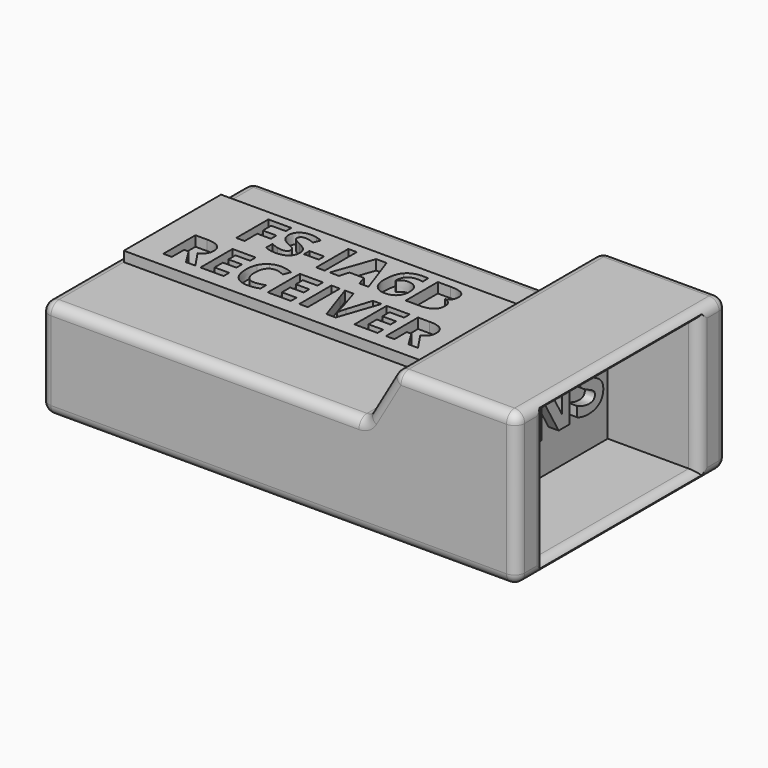
from build123d import *

# Parameters (mm, degrees)
F0_W          = 47
F0_H          = 15
F1_DEPTH      = 26
F3_DEPTH      = 26.001
F5_DEPTH      = 9
F6_TEXT_SIZE  = 6.9444444444
F7_DEPTH      = 1
F8_T1_DEPTH   = 26
F8_T3_DEPTH   = 30.4226497308
F8_T5_DEPTH   = 24
F8_T7_DEPTH   = 7.8038475773
F8_T9_DEPTH   = 13
F8_T11_DEPTH  = 45
F8_T13_DEPTH  = 4.8452994616
F8_T15_DEPTH  = 10.4226497308
F8_T17_DEPTH  = 19
F8_S21_W      = 1.02
F8_S21_H      = 1.02
F8_T22_DEPTH  = 1.02
F8_S27_W      = 1.02
F8_S27_H      = 1.02
F8_T28_DEPTH  = 1.02
F8_S33_W      = 1.02
F8_S33_H      = 1.02
F8_T34_DEPTH  = 1.02
F8_S39_W      = 1.02
F8_S39_H      = 1.02
F8_T40_DEPTH  = 1.02
F8_S45_W      = 1.02
F8_S45_H      = 1.02
F8_T46_DEPTH  = 1.02
F8_S51_W      = 1.02
F8_S51_H      = 1.02
F8_T52_DEPTH  = 1.02
F8_T58_DEPTH  = 1.02
F8_S63_W      = 1.02
F8_S63_H      = 1.02
F8_T64_DEPTH  = 1.02
F8_S69_W      = 1.02
F8_S69_H      = 1.02
F8_T70_DEPTH  = 1.02
F8_T76_DEPTH  = 1.02
F8_T80_ANGLE  = 60
F8_T82_ANGLE  = 60
F8_T87_DEPTH  = 21.5
F8_T91_DEPTH  = 15.5
F8_T99_DEPTH  = 21.5
F8_T103_DEPTH = 15.5
F8_T111_DEPTH = 15.5
F8_T116_DEPTH = 21.5
F8_T123_DEPTH = 21.5
F8_T127_DEPTH = 15.5
F9_W          = 0.8411458333
F9_H          = 3.9661458333
F9_W_2        = 1.4565972222
F9_H_2        = 0.6779513889
F10_DEPTH     = 1


# Not quite as in the source:
# - a fillet or chamfer that OpenCascade refuses, or shapes differently, is made with other operations: its cross-section is extruded or revolved along the edge and cut away or added
# - Text() gives the source's letters only with a copy of the font that has no kerning and outlines rounded to 1/6400 em; it was checked with that copy


with BuildPart() as f1:
    # F0 (on Front) → F1 (new body)
    with BuildSketch(Plane.XZ):
        with Locations((23.5, -7.5)):
            Rectangle(F0_W, F0_H)
    extrude(amount=F1_DEPTH)

    # F2 (on face) → F3 (cut, through all)
    with BuildSketch(Plane.XZ.offset(26)):
        Polygon((0, 0), (0, -5.1961524227), (32, -5.1961524227), (35, 0), align=None)
    extrude(amount=-F3_DEPTH, mode=Mode.SUBTRACT)

    # F4 (on face) → F5 (cut)
    with BuildSketch(Plane.YZ.offset(47)):
        Polygon((-16.9174801558, -1), (-22.5, -1), (-22.5, -9.4061652198), (-22.5, -14), (-8.8980188593, -14), (-3.5, -14), (-3.5, -5.7331291027), (-3.5, -1), align=None)
    extrude(amount=-F5_DEPTH, mode=Mode.SUBTRACT)

    # F8: fillet of radius 1 on 22 edges, made by hand

    # F8_s2 → F8_t1 (join)
    with BuildSketch(Plane.XZ):
        with BuildLine():
            ThreePointArc((32.2886751346, -4.6961524227), (31.9226497308, -5.0621778265), (31.4226497308, -5.1961524227))
            Line((31.4226497308, -5.1961524227), (32, -5.1961524227))
            Line((32, -5.1961524227), (32.2886751346, -4.6961524227))
        make_face()
    extrude(amount=F8_T1_DEPTH)

    # F8_s4 → F8_t3 (cut)
    with BuildSketch(Plane.YZ.offset(1)):
        with BuildLine():
            ThreePointArc((-26, -6.1961524227), (-25.7071067812, -5.4890456415), (-25, -5.1961524227))
            Line((-25, -5.1961524227), (-26, -5.1961524227))
            Line((-26, -5.1961524227), (-26, -6.1961524227))
        make_face()
        with BuildLine():
            ThreePointArc((0, -6.1961524227), (-0.2928932188, -5.4890456415), (-1, -5.1961524227))
            Line((-1, -5.1961524227), (0, -5.1961524227))
            Line((0, -5.1961524227), (0, -6.1961524227))
        make_face()
    extrude(amount=F8_T3_DEPTH, mode=Mode.SUBTRACT)

    # F8_s6 → F8_t5 (cut)
    with BuildSketch(Plane.XZ.offset(1)):
        with BuildLine():
            ThreePointArc((0, -6.1961524227), (0.2928932188, -5.4890456415), (1, -5.1961524227))
            Line((1, -5.1961524227), (0, -5.1961524227))
            Line((0, -5.1961524227), (0, -6.1961524227))
        make_face()
        with BuildLine():
            ThreePointArc((1, -15), (0.2928932188, -14.7071067812), (0, -14))
            Line((0, -14), (0, -15))
            Line((0, -15), (1, -15))
        make_face()
        with BuildLine():
            ThreePointArc((47, -14), (46.7071067812, -14.7071067812), (46, -15))
            Line((46, -15), (47, -15))
            Line((47, -15), (47, -14))
        make_face()
        with BuildLine():
            ThreePointArc((46, 0), (46.7071067812, -0.2928932188), (47, -1))
            Line((47, -1), (47, 0))
            Line((47, 0), (46, 0))
        make_face()
        with BuildLine():
            ThreePointArc((35.5773502692, 0), (35.0773502692, -0.1339745962), (34.7113248654, -0.5))
            Line((34.7113248654, -0.5), (35, 0))
            Line((35, 0), (35.5773502692, 0))
        make_face()
    extrude(amount=F8_T5_DEPTH, mode=Mode.SUBTRACT)

    # F8_s8 → F8_t7 (cut)
    with BuildSketch(Plane.XY.offset(-14)):
        with BuildLine():
            ThreePointArc((1, 0), (0.2928932188, -0.2928932188), (0, -1))
            Line((0, -1), (0, 0))
            Line((0, 0), (1, 0))
        make_face()
        with BuildLine():
            ThreePointArc((1, -26), (0.2928932188, -25.7071067812), (0, -25))
            Line((0, -25), (0, -26))
            Line((0, -26), (1, -26))
        make_face()
    extrude(amount=F8_T7_DEPTH, mode=Mode.SUBTRACT)

    # F8_s10 → F8_t9 (cut)
    with BuildSketch(Plane.XY.offset(-14)):
        with BuildLine():
            ThreePointArc((46, 0), (46.7071067812, -0.2928932188), (47, -1))
            Line((47, -1), (47, 0))
            Line((47, 0), (46, 0))
        make_face()
        with BuildLine():
            ThreePointArc((46, -26), (46.7071067812, -25.7071067812), (47, -25))
            Line((47, -25), (47, -26))
            Line((47, -26), (46, -26))
        make_face()
        with BuildLine():
            ThreePointArc((47, -2.5), (46.7071067812, -3.2071067812), (46, -3.5))
            Line((46, -3.5), (47, -3.5))
            Line((47, -3.5), (47, -2.5))
        make_face()
        with BuildLine():
            ThreePointArc((47, -23.5), (46.7071067812, -22.7928932188), (46, -22.5))
            Line((46, -22.5), (47, -22.5))
            Line((47, -22.5), (47, -23.5))
        make_face()
    extrude(amount=F8_T9_DEPTH, mode=Mode.SUBTRACT)

    # F8_s12 → F8_t11 (cut)
    with BuildSketch(Plane.YZ.offset(1)):
        with BuildLine():
            ThreePointArc((0, -14), (-0.2928932188, -14.7071067812), (-1, -15))
            Line((-1, -15), (0, -15))
            Line((0, -15), (0, -14))
        make_face()
        with BuildLine():
            ThreePointArc((-26, -14), (-25.7071067812, -14.7071067812), (-25, -15))
            Line((-25, -15), (-26, -15))
            Line((-26, -15), (-26, -14))
        make_face()
    extrude(amount=F8_T11_DEPTH, mode=Mode.SUBTRACT)

    # F8_s14 → F8_t13 (cut)
    with BuildSketch(Plane(origin=(6.0386751346, 0, 10.4592921435), x_dir=(0, 1, 0), z_dir=(0.5, 0, 0.8660254038))):
        with BuildLine():
            ThreePointArc((0, -31.3108891325), (-0.2928932188, -30.6037823513), (-1, -30.3108891325))
            Line((-1, -30.3108891325), (0, -30.3108891325))
            Line((0, -30.3108891325), (0, -31.3108891325))
        make_face()
        with BuildLine():
            ThreePointArc((-25, -30.3108891325), (-25.7071067812, -30.6037823513), (-26, -31.3108891325))
            Line((-26, -31.3108891325), (-26, -30.3108891325))
            Line((-26, -30.3108891325), (-25, -30.3108891325))
        make_face()
    extrude(amount=F8_T13_DEPTH, mode=Mode.SUBTRACT)

    # F8_s16 → F8_t15 (cut)
    with BuildSketch(Plane.YZ.offset(35.5773502692)):
        with BuildLine():
            ThreePointArc((-1, 0), (-0.2928932188, -0.2928932188), (0, -1))
            Line((0, -1), (0, 0))
            Line((0, 0), (-1, 0))
        make_face()
        with BuildLine():
            ThreePointArc((-25, 0), (-25.7071067812, -0.2928932188), (-26, -1))
            Line((-26, -1), (-26, 0))
            Line((-26, 0), (-25, 0))
        make_face()
    extrude(amount=F8_T15_DEPTH, mode=Mode.SUBTRACT)

    # F8_s18 → F8_t17 (cut)
    with BuildSketch(Plane.XZ.offset(3.5)):
        with BuildLine():
            ThreePointArc((47, 0), (46.7071067812, -0.7071067812), (46, -1))
            Line((46, -1), (47, -1))
            Line((47, -1), (47, 0))
        make_face()
        with BuildLine():
            ThreePointArc((47, -15), (46.7071067812, -14.2928932188), (46, -14))
            Line((46, -14), (47, -14))
            Line((47, -14), (47, -15))
        make_face()
    extrude(amount=F8_T17_DEPTH, mode=Mode.SUBTRACT)


with BuildPart() as f7:
    # F6 (on face) → F7 (new body)
    with BuildSketch(Plane.YZ.offset(38)):
        with Locations((-21.1532118056, -10)):
            Text('PINS', F6_TEXT_SIZE, font='Open Sans', font_style=FontStyle.BOLD, text_align=(TextAlign.LEFT, TextAlign.BOTTOM))
    extrude(amount=F7_DEPTH)


with BuildPart() as f8_tool20:
    # F8_s21 → F8_t22 (new body)
    with BuildSketch(Plane.XZ.offset(25)):
        with Locations((0.49, -5.6861524227)):
            Rectangle(F8_S21_W, F8_S21_H)
    extrude(amount=F8_T22_DEPTH)

    # F8_s23 → F8_t24 (revolve, cut)
    with BuildSketch(Plane(origin=(1, -25, -6.1961524227), x_dir=(0.7071067812, 0, -0.7071067812), z_dir=(-0.7071067812, 0, -0.7071067812))):
        with BuildLine():
            ThreePointArc((0, -1), (1, 0), (0, 1))
            Line((0, 1), (0, -1))
        make_face()
    revolve(axis=Axis((1, -25, -6.1961524227), (0, -1, 0)), mode=Mode.SUBTRACT)


with BuildPart() as f1_1:
    add(f1.part)

    # F8_t19: cut F8_tool20
    add(f8_tool20.part, mode=Mode.SUBTRACT)


with BuildPart() as f8_tool26:
    # F8_s27 → F8_t28 (new body)
    with BuildSketch(Plane.XZ.offset(1)):
        with Locations((0.49, -5.6861524227)):
            Rectangle(F8_S27_W, F8_S27_H)
    extrude(amount=-F8_T28_DEPTH)

    # F8_s29 → F8_t30 (revolve, cut)
    with BuildSketch(Plane(origin=(1, -1, -6.1961524227), x_dir=(0.7071067812, 0, -0.7071067812), z_dir=(0.7071067812, 0, 0.7071067812))):
        with BuildLine():
            ThreePointArc((0, -1), (1, 0), (0, 1))
            Line((0, 1), (0, -1))
        make_face()
    revolve(axis=Axis((1, -1, -6.1961524227), (0, 1, 0)), mode=Mode.SUBTRACT)


with BuildPart() as f1_2:
    add(f1_1.part)

    # F8_t25: cut F8_tool26
    add(f8_tool26.part, mode=Mode.SUBTRACT)


with BuildPart() as f8_tool32:
    # F8_s33 → F8_t34 (new body)
    with BuildSketch(Plane.XZ.offset(1)):
        with Locations((0.49, -14.51)):
            Rectangle(F8_S33_W, F8_S33_H)
    extrude(amount=-F8_T34_DEPTH)

    # F8_s35 → F8_t36 (revolve, cut)
    with BuildSketch(Plane(origin=(1, -1, -14), x_dir=(0.7071067812, 0, 0.7071067812), z_dir=(-0.7071067812, 0, 0.7071067812))):
        with BuildLine():
            ThreePointArc((0, -1), (1, 0), (0, 1))
            Line((0, 1), (0, -1))
        make_face()
    revolve(axis=Axis((1, -1, -14), (0, 1, 0)), mode=Mode.SUBTRACT)


with BuildPart() as f1_3:
    add(f1_2.part)

    # F8_t31: cut F8_tool32
    add(f8_tool32.part, mode=Mode.SUBTRACT)


with BuildPart() as f8_tool38:
    # F8_s39 → F8_t40 (new body)
    with BuildSketch(Plane.XZ.offset(25)):
        with Locations((0.49, -14.51)):
            Rectangle(F8_S39_W, F8_S39_H)
    extrude(amount=F8_T40_DEPTH)

    # F8_s41 → F8_t42 (revolve, cut)
    with BuildSketch(Plane(origin=(1, -25, -14), x_dir=(0.7071067812, 0, 0.7071067812), z_dir=(0.7071067812, 0, -0.7071067812))):
        with BuildLine():
            ThreePointArc((0, -1), (1, 0), (0, 1))
            Line((0, 1), (0, -1))
        make_face()
    revolve(axis=Axis((1, -25, -14), (0, -1, 0)), mode=Mode.SUBTRACT)


with BuildPart() as f1_4:
    add(f1_3.part)

    # F8_t37: cut F8_tool38
    add(f8_tool38.part, mode=Mode.SUBTRACT)


with BuildPart() as f8_tool44:
    # F8_s45 → F8_t46 (new body)
    with BuildSketch(Plane.XZ.offset(1)):
        with Locations((46.51, -14.51)):
            Rectangle(F8_S45_W, F8_S45_H)
    extrude(amount=-F8_T46_DEPTH)

    # F8_s47 → F8_t48 (revolve, cut)
    with BuildSketch(Plane(origin=(46, -1, -14), x_dir=(-0.7071067812, 0, 0.7071067812), z_dir=(-0.7071067812, 0, -0.7071067812))):
        with BuildLine():
            ThreePointArc((0, -1), (1, 0), (0, 1))
            Line((0, 1), (0, -1))
        make_face()
    revolve(axis=Axis((46, -1, -14), (0, 1, 0)), mode=Mode.SUBTRACT)


with BuildPart() as f1_5:
    add(f1_4.part)

    # F8_t43: cut F8_tool44
    add(f8_tool44.part, mode=Mode.SUBTRACT)


with BuildPart() as f8_tool50:
    # F8_s51 → F8_t52 (new body)
    with BuildSketch(Plane.XY.offset(-1)):
        with Locations((46.51, -0.49)):
            Rectangle(F8_S51_W, F8_S51_H)
    extrude(amount=F8_T52_DEPTH)

    # F8_s53 → F8_t54 (revolve, cut)
    with BuildSketch(Plane(origin=(46, -1, -1), x_dir=(-0.7071067812, -0.7071067812, 0), z_dir=(-0.7071067812, 0.7071067812, 0))):
        with BuildLine():
            ThreePointArc((0, -1), (1, 0), (0, 1))
            Line((0, 1), (0, -1))
        make_face()
    revolve(axis=Axis((46, -1, -1), (0, 0, 1)), mode=Mode.SUBTRACT)


with BuildPart() as f1_6:
    add(f1_5.part)

    # F8_t49: cut F8_tool50
    add(f8_tool50.part, mode=Mode.SUBTRACT)


with BuildPart() as f8_tool56:
    # F8_s57 → F8_t58 (new body)
    with BuildSketch(Plane.XZ.offset(1)):
        Polygon((35.5773502692, -1), (34.6940043573, -0.49), (34.9884529946, 0.02), (35.5773502692, 0.02), align=None)
    extrude(amount=-F8_T58_DEPTH)

    # F8_s59 → F8_t60 (revolve, cut)
    with BuildSketch(Plane(origin=(35.5773502692, -1, -1), x_dir=(0.5, 0, -0.8660254038), z_dir=(0.8660254038, 0, 0.5))):
        with BuildLine():
            ThreePointArc((0, -1), (1, 0), (0, 1))
            Line((0, 1), (0, -1))
        make_face()
    revolve(axis=Axis((35.5773502692, -1, -1), (0, 1, 0)), mode=Mode.SUBTRACT)


with BuildPart() as f1_7:
    add(f1_6.part)

    # F8_t55: cut F8_tool56
    add(f8_tool56.part, mode=Mode.SUBTRACT)


with BuildPart() as f8_tool62:
    # F8_s63 → F8_t64 (new body)
    with BuildSketch(Plane.XZ.offset(25)):
        with Locations((46.51, -14.51)):
            Rectangle(F8_S63_W, F8_S63_H)
    extrude(amount=F8_T64_DEPTH)

    # F8_s65 → F8_t66 (revolve, cut)
    with BuildSketch(Plane(origin=(46, -25, -14), x_dir=(-0.7071067812, 0, 0.7071067812), z_dir=(0.7071067812, 0, 0.7071067812))):
        with BuildLine():
            ThreePointArc((0, -1), (1, 0), (0, 1))
            Line((0, 1), (0, -1))
        make_face()
    revolve(axis=Axis((46, -25, -14), (0, -1, 0)), mode=Mode.SUBTRACT)


with BuildPart() as f1_8:
    add(f1_7.part)

    # F8_t61: cut F8_tool62
    add(f8_tool62.part, mode=Mode.SUBTRACT)


with BuildPart() as f8_tool68:
    # F8_s69 → F8_t70 (new body)
    with BuildSketch(Plane.XY.offset(-1)):
        with Locations((46.51, -25.51)):
            Rectangle(F8_S69_W, F8_S69_H)
    extrude(amount=F8_T70_DEPTH)

    # F8_s71 → F8_t72 (revolve, cut)
    with BuildSketch(Plane(origin=(46, -25, -1), x_dir=(-0.7071067812, 0.7071067812, 0), z_dir=(0.7071067812, 0.7071067812, 0))):
        with BuildLine():
            ThreePointArc((0, -1), (1, 0), (0, 1))
            Line((0, 1), (0, -1))
        make_face()
    revolve(axis=Axis((46, -25, -1), (0, 0, 1)), mode=Mode.SUBTRACT)


with BuildPart() as f1_9:
    add(f1_8.part)

    # F8_t67: cut F8_tool68
    add(f8_tool68.part, mode=Mode.SUBTRACT)


with BuildPart() as f8_tool74:
    # F8_s75 → F8_t76 (new body)
    with BuildSketch(Plane.XZ.offset(25)):
        Polygon((35.5773502692, -1), (35.5773502692, 0.02), (34.9884529946, 0.02), (34.6940043573, -0.49), align=None)
    extrude(amount=F8_T76_DEPTH)

    # F8_s77 → F8_t78 (revolve, cut)
    with BuildSketch(Plane(origin=(35.5773502692, -25, -1), x_dir=(0.5, 0, -0.8660254038), z_dir=(-0.8660254038, 0, -0.5))):
        with BuildLine():
            ThreePointArc((0, -1), (1, 0), (0, 1))
            Line((0, 1), (0, -1))
        make_face()
    revolve(axis=Axis((35.5773502692, -25, -1), (0, -1, 0)), mode=Mode.SUBTRACT)


with BuildPart() as f1_10:
    add(f1_9.part)

    # F8_t73: cut F8_tool74
    add(f8_tool74.part, mode=Mode.SUBTRACT)

    # F8_s79 → F8_t80 (revolve, cut)
    with BuildSketch(Plane(origin=(6.0386751346, 0, 10.4592921435), x_dir=(0, 1, 0), z_dir=(0.5, 0, 0.8660254038))):
        with BuildLine():
            ThreePointArc((-26, -31.3108891325), (-25.7071067812, -30.6037823513), (-25, -30.3108891325))
            Line((-25, -30.3108891325), (-26, -30.3108891325))
            Line((-26, -30.3108891325), (-26, -31.3108891325))
        make_face()
    revolve(axis=Axis((31.4226497308, -26, -4.1961524227), (0, 1, 0)), revolution_arc=F8_T80_ANGLE, mode=Mode.SUBTRACT)

    # F8_s81 → F8_t82 (revolve, cut)
    with BuildSketch(Plane(origin=(6.0386751346, 0, 10.4592921435), x_dir=(0, 1, 0), z_dir=(0.5, 0, 0.8660254038))):
        with BuildLine():
            ThreePointArc((0, -31.3108891325), (-0.2928932188, -30.6037823513), (-1, -30.3108891325))
            Line((-1, -30.3108891325), (0, -30.3108891325))
            Line((0, -30.3108891325), (0, -31.3108891325))
        make_face()
    revolve(axis=Axis((31.4226497308, 0, -4.1961524227), (0, 1, 0)), revolution_arc=F8_T82_ANGLE, mode=Mode.SUBTRACT)


with BuildPart() as f8_tool85:
    # F8_s86 → F8_t87 (new body)
    with BuildSketch(Plane.XZ.offset(25)):
        with BuildLine():
            ThreePointArc((47, 0), (46.7071067812, -0.7071067812), (46, -1))
            Line((46, -1), (47, -1))
            Line((47, -1), (47, 0))
        make_face()
    extrude(amount=-F8_T87_DEPTH)

    split(bisect_by=Plane.XZ.offset(22.5), keep=Keep.TOP)


with BuildPart() as f8_tool89:
    # F8_s90 → F8_t91 (new body)
    with BuildSketch(Plane.XY.offset(-14)):
        with BuildLine():
            ThreePointArc((47, -23.5), (46.7071067812, -22.7928932188), (46, -22.5))
            Line((46, -22.5), (47, -22.5))
            Line((47, -22.5), (47, -23.5))
        make_face()
    extrude(amount=F8_T91_DEPTH)

    split(bisect_by=Plane.XY, keep=Keep.BOTTOM)

    split(bisect_by=Plane.XY.offset(-1), keep=Keep.TOP)


with BuildPart() as f8_tool85_1:
    add(f8_tool85.part)

    # F8_t94: intersect F8_tool89
    add(f8_tool89.part, mode=Mode.INTERSECT)


with BuildPart() as f1_11:
    add(f1_10.part)

    # F8_t83: cut F8_tool85
    add(f8_tool85_1.part, mode=Mode.SUBTRACT)


with BuildPart() as f8_tool97:
    # F8_s98 → F8_t99 (new body)
    with BuildSketch(Plane.XZ.offset(22.5)):
        with BuildLine():
            ThreePointArc((47, 0), (46.7071067812, -0.7071067812), (46, -1))
            Line((46, -1), (47, -1))
            Line((47, -1), (47, 0))
        make_face()
    extrude(amount=-F8_T99_DEPTH)

    split(bisect_by=Plane.XZ.offset(3.5), keep=Keep.BOTTOM)


with BuildPart() as f8_tool101:
    # F8_s102 → F8_t103 (new body)
    with BuildSketch(Plane.XY.offset(1.5)):
        with BuildLine():
            ThreePointArc((47, -2.5), (46.7071067812, -3.2071067812), (46, -3.5))
            Line((46, -3.5), (47, -3.5))
            Line((47, -3.5), (47, -2.5))
        make_face()
    extrude(amount=-F8_T103_DEPTH)

    split(bisect_by=Plane.XY, keep=Keep.BOTTOM)

    split(bisect_by=Plane.XY.offset(-1), keep=Keep.TOP)


with BuildPart() as f8_tool97_1:
    add(f8_tool97.part)

    # F8_t106: intersect F8_tool101
    add(f8_tool101.part, mode=Mode.INTERSECT)


with BuildPart() as f1_12:
    add(f1_11.part)

    # F8_t95: cut F8_tool97
    add(f8_tool97_1.part, mode=Mode.SUBTRACT)


with BuildPart() as f8_tool109:
    # F8_s110 → F8_t111 (new body)
    with BuildSketch(Plane.XY.offset(-1)):
        with BuildLine():
            ThreePointArc((47, -2.5), (46.7071067812, -3.2071067812), (46, -3.5))
            Line((46, -3.5), (47, -3.5))
            Line((47, -3.5), (47, -2.5))
        make_face()
    extrude(amount=-F8_T111_DEPTH)

    split(bisect_by=Plane.XY.offset(-15), keep=Keep.TOP)

    split(bisect_by=Plane.XY.offset(-14), keep=Keep.BOTTOM)


with BuildPart() as f8_tool114:
    # F8_s115 → F8_t116 (new body)
    with BuildSketch(Plane.XZ.offset(1)):
        with BuildLine():
            ThreePointArc((47, -15), (46.7071067812, -14.2928932188), (46, -14))
            Line((46, -14), (47, -14))
            Line((47, -14), (47, -15))
        make_face()
    extrude(amount=F8_T116_DEPTH)

    split(bisect_by=Plane.XZ.offset(3.5), keep=Keep.BOTTOM)


with BuildPart() as f8_tool109_1:
    add(f8_tool109.part)

    # F8_t118: intersect F8_tool114
    add(f8_tool114.part, mode=Mode.INTERSECT)


with BuildPart() as f1_13:
    add(f1_12.part)

    # F8_t107: cut F8_tool109
    add(f8_tool109_1.part, mode=Mode.SUBTRACT)


with BuildPart() as f8_tool121:
    # F8_s122 → F8_t123 (new body)
    with BuildSketch(Plane.XZ.offset(3.5)):
        with BuildLine():
            ThreePointArc((47, -15), (46.7071067812, -14.2928932188), (46, -14))
            Line((46, -14), (47, -14))
            Line((47, -14), (47, -15))
        make_face()
    extrude(amount=F8_T123_DEPTH)

    split(bisect_by=Plane.XZ.offset(22.5), keep=Keep.TOP)


with BuildPart() as f8_tool125:
    # F8_s126 → F8_t127 (new body)
    with BuildSketch(Plane.XY.offset(-16.5)):
        with BuildLine():
            ThreePointArc((47, -23.5), (46.7071067812, -22.7928932188), (46, -22.5))
            Line((46, -22.5), (47, -22.5))
            Line((47, -22.5), (47, -23.5))
        make_face()
    extrude(amount=F8_T127_DEPTH)

    split(bisect_by=Plane.XY.offset(-15), keep=Keep.TOP)

    split(bisect_by=Plane.XY.offset(-14), keep=Keep.BOTTOM)


with BuildPart() as f8_tool121_1:
    add(f8_tool121.part)

    # F8_t130: intersect F8_tool125
    add(f8_tool125.part, mode=Mode.INTERSECT)


with BuildPart() as f1_14:
    add(f1_13.part)

    # F8_t119: cut F8_tool121
    add(f8_tool121_1.part, mode=Mode.SUBTRACT)


with BuildPart() as f10:
    # F9 (on face) → F10 (new body)
    with BuildSketch(Plane.XY.offset(-5.1961524227)):
        Polygon((1, -17), (18.8139621168, -17), (31.4226497308, -17), (31.4226497308, -13.5022401258), (31.4226497308, -7.9219900222), (31.4226497308, -5), (20.9267525453, -5), (1, -5), (1, -7.9219900222), (1, -15.4874399304), align=None)
        with BuildLine():
            Line((4.989536671, -13.9805387369), (4.5424880598, -13.9805387369))
            Line((4.5424880598, -13.9805387369), (4.5424880598, -15.5022401258))
            Line((4.5424880598, -15.5022401258), (3.7013422265, -15.5022401258))
            Line((3.7013422265, -15.5022401258), (3.7013422265, -11.5360942925))
            Line((3.7013422265, -11.5360942925), (4.856724171, -11.5360942925))
            add(Edge.make_bspline(
                [(4.856724171, -11.5360942925), (5.6657519487, -11.5360942925), (6.0533387543, -11.8303651258)],
                knots=[0, 0, 0, 1, 1, 1], degree=2))
            add(Edge.make_bspline(
                [(6.0533387543, -11.8303651258), (6.4409255598, -12.1246359591), (6.4409255598, -12.724462348)],
                knots=[0, 0, 0, 1, 1, 1], degree=2))
            add(Edge.make_bspline(
                [(6.4409255598, -12.724462348), (6.4409255598, -13.0742887369), (6.2486512543, -13.3468581813)],
                knots=[0, 0, 0, 1, 1, 1], degree=2))
            add(Edge.make_bspline(
                [(6.2486512543, -13.3468581813), (6.0563769487, -13.6194276258), (5.7030783376, -13.7739415147)],
                knots=[0, 0, 0, 1, 1, 1], degree=2))
            add(Edge.make_bspline(
                [(5.7030783376, -13.7739415147), (6.598911671, -15.1116151258), (6.8697450043, -15.5022401258)],
                knots=[0, 0, 0, 1, 1, 1], degree=2))
            Line((6.8697450043, -15.5022401258), (5.9365852821, -15.5022401258))
            Line((5.9365852821, -15.5022401258), (4.989536671, -13.9805387369))
        make_face(mode=Mode.SUBTRACT)
        Polygon((9.6527311154, -14.8077956813), (9.6527311154, -15.5022401258), (7.3688769487, -15.5022401258), (7.3688769487, -11.5360942925), (9.6527311154, -11.5360942925), (9.6527311154, -12.2253304036), (8.2100227821, -12.2253304036), (8.2100227821, -13.0959901258), (9.5529047265, -13.0959901258), (9.5529047265, -13.7852262369), (8.2100227821, -13.7852262369), (8.2100227821, -14.8077956813), align=None, mode=Mode.SUBTRACT)
        with BuildLine():
            add(Edge.make_bspline(
                [(12.606724171, -12.2578824869), (12.3818977821, -12.1793234591), (12.1648838932, -12.1793234591)],
                knots=[0, 0, 0, 1, 1, 1], degree=2))
            add(Edge.make_bspline(
                [(12.1648838932, -12.1793234591), (11.6900575043, -12.1793234591), (11.4296408376, -12.5360942925)],
                knots=[0, 0, 0, 1, 1, 1], degree=2))
            add(Edge.make_bspline(
                [(11.4296408376, -12.5360942925), (11.169224171, -12.8928651258), (11.169224171, -13.5300179036)],
                knots=[0, 0, 0, 1, 1, 1], degree=2))
            add(Edge.make_bspline(
                [(11.169224171, -13.5300179036), (11.169224171, -14.8564067925), (12.1648838932, -14.8564067925)],
                knots=[0, 0, 0, 1, 1, 1], degree=2))
            add(Edge.make_bspline(
                [(12.1648838932, -14.8564067925), (12.5824186154, -14.8564067925), (13.1761686154, -14.6480734591)],
                knots=[0, 0, 0, 1, 1, 1], degree=2))
            Line((13.1761686154, -14.6480734591), (13.1761686154, -15.3529345702))
            add(Edge.make_bspline(
                [(13.1761686154, -15.3529345702), (12.6883213932, -15.5569276258), (12.0858908376, -15.5569276258)],
                knots=[0, 0, 0, 1, 1, 1], degree=2))
            add(Edge.make_bspline(
                [(12.0858908376, -15.5569276258), (11.2204394487, -15.5569276258), (10.7621061154, -15.0317540147)],
                knots=[0, 0, 0, 1, 1, 1], degree=2))
            add(Edge.make_bspline(
                [(10.7621061154, -15.0317540147), (10.3037727821, -14.5065804036), (10.3037727821, -13.5248095702)],
                knots=[0, 0, 0, 1, 1, 1], degree=2))
            add(Edge.make_bspline(
                [(10.3037727821, -13.5248095702), (10.3037727821, -12.9058859591), (10.5290331987, -12.4406081813)],
                knots=[0, 0, 0, 1, 1, 1], degree=2))
            add(Edge.make_bspline(
                [(10.5290331987, -12.4406081813), (10.7542936154, -11.9753304036), (11.1761686154, -11.7275005425)],
                knots=[0, 0, 0, 1, 1, 1], degree=2))
            add(Edge.make_bspline(
                [(11.1761686154, -11.7275005425), (11.5980436154, -11.4796706813), (12.1648838932, -11.4796706813)],
                knots=[0, 0, 0, 1, 1, 1], degree=2))
            add(Edge.make_bspline(
                [(12.1648838932, -11.4796706813), (12.7421408376, -11.4796706813), (13.325474171, -11.7583165147)],
                knots=[0, 0, 0, 1, 1, 1], degree=2))
            Line((13.325474171, -11.7583165147), (13.0546408376, -12.4423442925))
            add(Edge.make_bspline(
                [(13.0546408376, -12.4423442925), (12.8315505598, -12.3364415147), (12.606724171, -12.2578824869)],
                knots=[0, 0, 0, 1, 1, 1], degree=2))
        make_face(mode=Mode.SUBTRACT)
        Polygon((16.3037727821, -14.8077956813), (16.3037727821, -15.5022401258), (14.0199186154, -15.5022401258), (14.0199186154, -11.5360942925), (16.3037727821, -11.5360942925), (16.3037727821, -12.2253304036), (14.8610644487, -12.2253304036), (14.8610644487, -13.0959901258), (16.2039463932, -13.0959901258), (16.2039463932, -13.7852262369), (14.8610644487, -13.7852262369), (14.8610644487, -14.8077956813), align=None, mode=Mode.SUBTRACT)
        with Locations((17.5516026432, -13.5191672091)):
            Rectangle(F9_W, F9_H, mode=Mode.SUBTRACT)
        with BuildLine():
            Line((18.4713075043, -11.5360942925), (18.8139621168, -11.5360942925))
            Line((18.8139621168, -11.5360942925), (19.3202658376, -11.5360942925))
            Line((19.3202658376, -11.5360942925), (20.0667936154, -13.896337348))
            add(Edge.make_bspline(
                [(20.0667936154, -13.896337348), (20.1284255598, -14.1055387369), (20.1952658376, -14.3833165147)],
                knots=[0, 0, 0, 1, 1, 1], degree=2))
            add(Edge.make_bspline(
                [(20.1952658376, -14.3833165147), (20.2621061154, -14.6610942925), (20.2777311154, -14.7696012369)],
                knots=[0, 0, 0, 1, 1, 1], degree=2))
            add(Edge.make_bspline(
                [(20.2777311154, -14.7696012369), (20.3081130598, -14.5204692925), (20.481724171, -13.896337348)],
                knots=[0, 0, 0, 1, 1, 1], degree=2))
            Line((20.481724171, -13.896337348), (21.2325922265, -11.5360942925))
            Line((21.2325922265, -11.5360942925), (22.0815505598, -11.5360942925))
            Line((22.0815505598, -11.5360942925), (20.7334602821, -15.5022401258))
            Line((20.7334602821, -15.5022401258), (19.8167936154, -15.5022401258))
            Line((19.8167936154, -15.5022401258), (18.8139621168, -12.5461516632))
            Line((18.8139621168, -12.5461516632), (18.4713075043, -11.5360942925))
        make_face(mode=Mode.SUBTRACT)
        Polygon((24.864536671, -14.8077956813), (24.864536671, -15.5022401258), (22.5806825043, -15.5022401258), (22.5806825043, -11.5360942925), (24.864536671, -11.5360942925), (24.864536671, -12.2253304036), (23.4218283376, -12.2253304036), (23.4218283376, -13.0959901258), (24.7647102821, -13.0959901258), (24.7647102821, -13.7852262369), (23.4218283376, -13.7852262369), (23.4218283376, -14.8077956813), align=None, mode=Mode.SUBTRACT)
        with BuildLine():
            Line((26.9799880598, -13.9805387369), (26.5329394487, -13.9805387369))
            Line((26.5329394487, -13.9805387369), (26.5329394487, -15.5022401258))
            Line((26.5329394487, -15.5022401258), (25.6917936154, -15.5022401258))
            Line((25.6917936154, -15.5022401258), (25.6917936154, -11.5360942925))
            Line((25.6917936154, -11.5360942925), (26.8471755598, -11.5360942925))
            add(Edge.make_bspline(
                [(26.8471755598, -11.5360942925), (27.6562033376, -11.5360942925), (28.0437901432, -11.8303651258)],
                knots=[0, 0, 0, 1, 1, 1], degree=2))
            add(Edge.make_bspline(
                [(28.0437901432, -11.8303651258), (28.4313769487, -12.1246359591), (28.4313769487, -12.724462348)],
                knots=[0, 0, 0, 1, 1, 1], degree=2))
            add(Edge.make_bspline(
                [(28.4313769487, -12.724462348), (28.4313769487, -13.0742887369), (28.2391026432, -13.3468581813)],
                knots=[0, 0, 0, 1, 1, 1], degree=2))
            add(Edge.make_bspline(
                [(28.2391026432, -13.3468581813), (28.0468283376, -13.6194276258), (27.6935297265, -13.7739415147)],
                knots=[0, 0, 0, 1, 1, 1], degree=2))
            add(Edge.make_bspline(
                [(27.6935297265, -13.7739415147), (28.5893630598, -15.1116151258), (28.8601963932, -15.5022401258)],
                knots=[0, 0, 0, 1, 1, 1], degree=2))
            Line((28.8601963932, -15.5022401258), (27.927036671, -15.5022401258))
            Line((27.927036671, -15.5022401258), (26.9799880598, -13.9805387369))
        make_face(mode=Mode.SUBTRACT)
        with Locations((12.9443977821, -8.4328407167)):
            Rectangle(F9_W_2, F9_H_2, mode=Mode.SUBTRACT)
        Polygon((7.2673144487, -8.3542816889), (7.2673144487, -9.9219900222), (6.4400575043, -9.9219900222), (6.4400575043, -5.9558441889), (8.7134950043, -5.9558441889), (8.7134950043, -6.6450803), (7.2673144487, -6.6450803), (7.2673144487, -7.6676497445), (8.6128005598, -7.6676497445), (8.6128005598, -8.3542816889), align=None, mode=Mode.SUBTRACT)
        with BuildLine():
            add(Edge.make_bspline(
                [(11.6245193098, -8.1654796056), (11.8306825043, -8.4324066889), (11.8306825043, -8.8204275222)],
                knots=[0, 0, 0, 1, 1, 1], degree=2))
            add(Edge.make_bspline(
                [(11.8306825043, -8.8204275222), (11.8306825043, -9.3577539111), (11.4439637543, -9.6672157167)],
                knots=[0, 0, 0, 1, 1, 1], degree=2))
            add(Edge.make_bspline(
                [(11.4439637543, -9.6672157167), (11.0572450043, -9.9766775222), (10.3688769487, -9.9766775222)],
                knots=[0, 0, 0, 1, 1, 1], degree=2))
            add(Edge.make_bspline(
                [(10.3688769487, -9.9766775222), (9.7334602821, -9.9766775222), (9.2456130598, -9.7370941889)],
                knots=[0, 0, 0, 1, 1, 1], degree=2))
            Line((9.2456130598, -9.7370941889), (9.2456130598, -8.9558441889))
            add(Edge.make_bspline(
                [(9.2456130598, -8.9558441889), (9.6466547265, -9.1355316889), (9.9248665321, -9.2084483556)],
                knots=[0, 0, 0, 1, 1, 1], degree=2))
            add(Edge.make_bspline(
                [(9.9248665321, -9.2084483556), (10.2030783376, -9.2813650222), (10.4339811154, -9.2813650222)],
                knots=[0, 0, 0, 1, 1, 1], degree=2))
            add(Edge.make_bspline(
                [(10.4339811154, -9.2813650222), (10.7100227821, -9.2813650222), (10.8580262543, -9.1758962722)],
                knots=[0, 0, 0, 1, 1, 1], degree=2))
            add(Edge.make_bspline(
                [(10.8580262543, -9.1758962722), (11.0060297265, -9.0704275222), (11.0060297265, -8.8612261334)],
                knots=[0, 0, 0, 1, 1, 1], degree=2))
            add(Edge.make_bspline(
                [(11.0060297265, -8.8612261334), (11.0060297265, -8.7449066889), (10.9409255598, -8.6537608556)],
                knots=[0, 0, 0, 1, 1, 1], degree=2))
            add(Edge.make_bspline(
                [(10.9409255598, -8.6537608556), (10.8758213932, -8.5626150222), (10.7495193098, -8.4788476611)],
                knots=[0, 0, 0, 1, 1, 1], degree=2))
            add(Edge.make_bspline(
                [(10.7495193098, -8.4788476611), (10.6232172265, -8.3950803), (10.2351963932, -8.2101844667)],
                knots=[0, 0, 0, 1, 1, 1], degree=2))
            add(Edge.make_bspline(
                [(10.2351963932, -8.2101844667), (9.872349171, -8.0391775222), (9.6904915321, -7.8820594667)],
                knots=[0, 0, 0, 1, 1, 1], degree=2))
            add(Edge.make_bspline(
                [(9.6904915321, -7.8820594667), (9.5086338932, -7.7249414111), (9.4001269487, -7.5157400222)],
                knots=[0, 0, 0, 1, 1, 1], degree=2))
            add(Edge.make_bspline(
                [(9.4001269487, -7.5157400222), (9.2916200043, -7.3065386334), (9.2916200043, -7.0278928)],
                knots=[0, 0, 0, 1, 1, 1], degree=2))
            add(Edge.make_bspline(
                [(9.2916200043, -7.0278928), (9.2916200043, -6.5009830778), (9.6483908376, -6.2002018278)],
                knots=[0, 0, 0, 1, 1, 1], degree=2))
            add(Edge.make_bspline(
                [(9.6483908376, -6.2002018278), (10.005161671, -5.8994205778), (10.6345019487, -5.8994205778)],
                knots=[0, 0, 0, 1, 1, 1], degree=2))
            add(Edge.make_bspline(
                [(10.6345019487, -5.8994205778), (10.9435297265, -5.8994205778), (11.2243456987, -5.9723372445)],
                knots=[0, 0, 0, 1, 1, 1], degree=2))
            add(Edge.make_bspline(
                [(11.2243456987, -5.9723372445), (11.505161671, -6.0452539111), (11.8115852821, -6.1780664111)],
                knots=[0, 0, 0, 1, 1, 1], degree=2))
            Line((11.8115852821, -6.1780664111), (11.5407519487, -6.8325803))
            add(Edge.make_bspline(
                [(11.5407519487, -6.8325803), (11.2230436154, -6.7023719667), (11.0155783376, -6.6507226611)],
                knots=[0, 0, 0, 1, 1, 1], degree=2))
            add(Edge.make_bspline(
                [(11.0155783376, -6.6507226611), (10.8081130598, -6.5990733556), (10.6075922265, -6.5990733556)],
                knots=[0, 0, 0, 1, 1, 1], degree=2))
            add(Edge.make_bspline(
                [(10.6075922265, -6.5990733556), (10.3688769487, -6.5990733556), (10.2412727821, -6.7101844667)],
                knots=[0, 0, 0, 1, 1, 1], degree=2))
            add(Edge.make_bspline(
                [(10.2412727821, -6.7101844667), (10.1136686154, -6.8212955778), (10.1136686154, -7.0001150222)],
                knots=[0, 0, 0, 1, 1, 1], degree=2))
            add(Edge.make_bspline(
                [(10.1136686154, -7.0001150222), (10.1136686154, -7.1112261334), (10.165317921, -7.1941254389)],
                knots=[0, 0, 0, 1, 1, 1], degree=2))
            add(Edge.make_bspline(
                [(10.165317921, -7.1941254389), (10.2169672265, -7.2770247445), (10.329380421, -7.3542816889)],
                knots=[0, 0, 0, 1, 1, 1], degree=2))
            add(Edge.make_bspline(
                [(10.329380421, -7.3542816889), (10.4417936154, -7.4315386334), (10.8619325043, -7.6320594667)],
                knots=[0, 0, 0, 1, 1, 1], degree=2))
            add(Edge.make_bspline(
                [(10.8619325043, -7.6320594667), (11.4183561154, -7.8985525222), (11.6245193098, -8.1654796056)],
                knots=[0, 0, 0, 1, 1, 1], degree=2))
        make_face(mode=Mode.SUBTRACT)
        with Locations((14.7573318098, -7.9389171056)):
            Rectangle(F9_W, F9_H, mode=Mode.SUBTRACT)
        Polygon((19.5103700043, -9.9219900222), (18.8139621168, -9.9219900222), (18.6041200043, -9.9219900222), (18.3167936154, -8.9775455778), (16.8706130598, -8.9775455778), (16.583286671, -9.9219900222), (15.677036671, -9.9219900222), (17.0772102821, -5.9393511334), (18.1049880598, -5.9393511334), align=None, mode=Mode.SUBTRACT)
        with BuildLine():
            add(Edge.make_bspline(
                [(19.8831998654, -9.1789344667), (19.7056825043, -8.7883094667), (19.7056825043, -8.2370941889)],
                knots=[0, 0, 0, 1, 1, 1], degree=2))
            add(Edge.make_bspline(
                [(19.7056825043, -8.2370941889), (19.7056825043, -7.0600108556), (20.2035123654, -6.48492405)],
                knots=[0, 0, 0, 1, 1, 1], degree=2))
            add(Edge.make_bspline(
                [(20.2035123654, -6.48492405), (20.7013422265, -5.9098372445), (21.6943977821, -5.9098372445)],
                knots=[0, 0, 0, 1, 1, 1], degree=2))
            add(Edge.make_bspline(
                [(21.6943977821, -5.9098372445), (22.0329394487, -5.9098372445), (22.2256477821, -5.9506358556)],
                knots=[0, 0, 0, 1, 1, 1], degree=2))
            Line((22.2256477821, -5.9506358556), (22.2256477821, -6.6207747445))
            add(Edge.make_bspline(
                [(22.2256477821, -6.6207747445), (21.9843283376, -6.5660872445), (21.7482172265, -6.5660872445)],
                knots=[0, 0, 0, 1, 1, 1], degree=2))
            add(Edge.make_bspline(
                [(21.7482172265, -6.5660872445), (21.3167936154, -6.5660872445), (21.044224171, -6.6962955778)],
                knots=[0, 0, 0, 1, 1, 1], degree=2))
            add(Edge.make_bspline(
                [(21.044224171, -6.6962955778), (20.7716547265, -6.8265039111), (20.6362380598, -7.0817122445)],
                knots=[0, 0, 0, 1, 1, 1], degree=2))
            add(Edge.make_bspline(
                [(20.6362380598, -7.0817122445), (20.5008213932, -7.3369205778), (20.4765158376, -7.8056705778)],
                knots=[0, 0, 0, 1, 1, 1], degree=2))
            Line((20.4765158376, -7.8056705778), (20.5112380598, -7.8056705778))
            add(Edge.make_bspline(
                [(20.5112380598, -7.8056705778), (20.7803352821, -7.3447330778), (21.3714811154, -7.3447330778)],
                knots=[0, 0, 0, 1, 1, 1], degree=2))
            add(Edge.make_bspline(
                [(21.3714811154, -7.3447330778), (21.9027311154, -7.3447330778), (22.2039463932, -7.6785004389)],
                knots=[0, 0, 0, 1, 1, 1], degree=2))
            add(Edge.make_bspline(
                [(22.2039463932, -7.6785004389), (22.505161671, -8.0122678), (22.505161671, -8.6008094667)],
                knots=[0, 0, 0, 1, 1, 1], degree=2))
            add(Edge.make_bspline(
                [(22.505161671, -8.6008094667), (22.505161671, -9.2353580778), (22.1470887543, -9.6060178)],
                knots=[0, 0, 0, 1, 1, 1], degree=2))
            add(Edge.make_bspline(
                [(22.1470887543, -9.6060178), (21.7890158376, -9.9766775222), (21.1544672265, -9.9766775222)],
                knots=[0, 0, 0, 1, 1, 1], degree=2))
            add(Edge.make_bspline(
                [(21.1544672265, -9.9766775222), (20.7152311154, -9.9766775222), (20.387974171, -9.7731184945)],
                knots=[0, 0, 0, 1, 1, 1], degree=2))
            add(Edge.make_bspline(
                [(20.387974171, -9.7731184945), (20.0607172265, -9.5695594667), (19.8831998654, -9.1789344667)],
                knots=[0, 0, 0, 1, 1, 1], degree=2))
        make_face(mode=Mode.SUBTRACT)
        with BuildLine():
            Line((23.1805088932, -9.9219900222), (23.1805088932, -5.9558441889))
            Line((23.1805088932, -5.9558441889), (24.4148838932, -5.9558441889))
            add(Edge.make_bspline(
                [(24.4148838932, -5.9558441889), (25.2586338932, -5.9558441889), (25.6397102821, -6.19586155)],
                knots=[0, 0, 0, 1, 1, 1], degree=2))
            add(Edge.make_bspline(
                [(25.6397102821, -6.19586155), (26.020786671, -6.4358789111), (26.020786671, -6.9593164111)],
                knots=[0, 0, 0, 1, 1, 1], degree=2))
            add(Edge.make_bspline(
                [(26.020786671, -6.9593164111), (26.020786671, -7.3152191889), (25.8541200043, -7.5430837722)],
                knots=[0, 0, 0, 1, 1, 1], degree=2))
            add(Edge.make_bspline(
                [(25.8541200043, -7.5430837722), (25.6874533376, -7.7709483556), (25.4105436154, -7.8169553)],
                knots=[0, 0, 0, 1, 1, 1], degree=2))
            Line((25.4105436154, -7.8169553), (25.4105436154, -7.8438650222))
            add(Edge.make_bspline(
                [(25.4105436154, -7.8438650222), (25.7872797265, -7.9280664111), (25.954380421, -8.1585351611)],
                knots=[0, 0, 0, 1, 1, 1], degree=2))
            add(Edge.make_bspline(
                [(25.954380421, -8.1585351611), (26.1214811154, -8.3890039111), (26.1214811154, -8.7718164111)],
                knots=[0, 0, 0, 1, 1, 1], degree=2))
            add(Edge.make_bspline(
                [(26.1214811154, -8.7718164111), (26.1214811154, -9.3143511334), (25.7291200043, -9.6181705778)],
                knots=[0, 0, 0, 1, 1, 1], degree=2))
            add(Edge.make_bspline(
                [(25.7291200043, -9.6181705778), (25.3367588932, -9.9219900222), (24.6640158376, -9.9219900222)],
                knots=[0, 0, 0, 1, 1, 1], degree=2))
            Line((24.6640158376, -9.9219900222), (23.1805088932, -9.9219900222))
        make_face(mode=Mode.SUBTRACT)
    extrude(amount=F10_DEPTH)


solid = Compound([f7.part, f1_14.part, f10.part])
